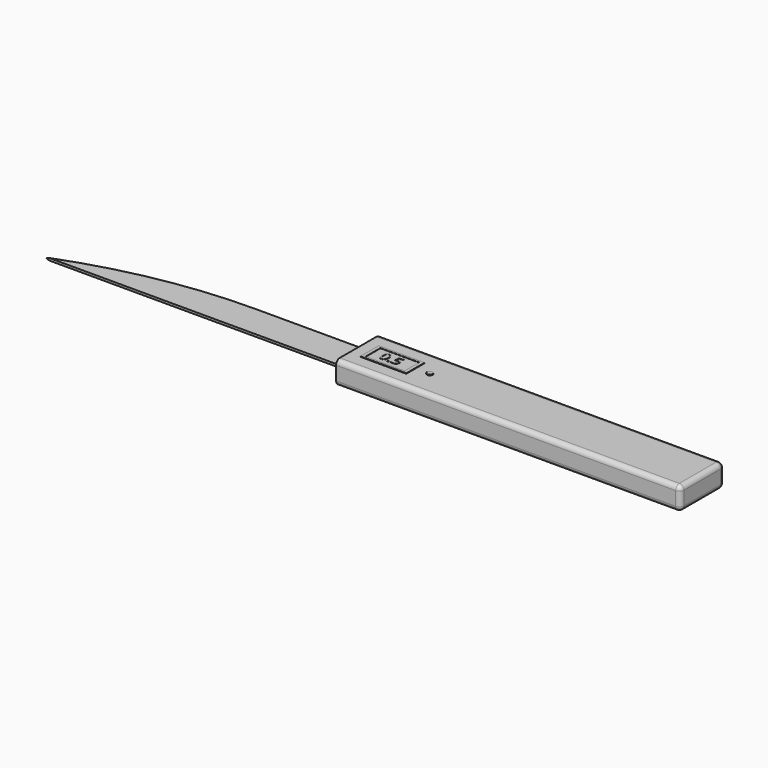
from build123d import *

# Parameters (mm, degrees)
F0_W          = 190.5
F0_H          = 30.48
F1_DEPTH      = 6.35
F1_DEPTH_BACK = 6.35
F3_DEPTH      = 0.635
F3_DEPTH_BACK = 0.635
F4_R          = 2.54
F5_SIZE       = 0.63499
F6_W          = 25.4
F6_H          = 12.7
F7_DEPTH      = 0.254
F8_R          = 1.5875
F9_DEPTH      = 0.381
F10_R         = 0.127
F11_W         = 21.59
F11_H         = 10.16
F12_DEPTH     = 0.127
F13_TEXT_SIZE = 7.8455061343
F14_DEPTH     = 0.127


# Not quite as in the source:
# - a fillet or chamfer is up to 0.001 mm smaller than in the source, because OpenCascade refuses the exact size
# - Text() gives the source's letters only with a copy of the font that has no kerning and outlines rounded to 1/6400 em; it was checked with that copy


with BuildPart() as f1:
    # F0 (on Top) → F1 (new body, two sides)
    with BuildSketch(Plane.XY) as f1_sk:
        with Locations((95.25, 0)):
            Rectangle(F0_W, F0_H)
    extrude(amount=F1_DEPTH)
    extrude(f1_sk.sketch, amount=-F1_DEPTH_BACK)

    # F4
    f4_edges = [f1.edges().sort_by_distance(p)[0] for p in [
        (95.25, -15.24, 6.35),
        (95.25, -15.24, -6.35),
        (190.5, -15.24, 0),
        (190.5, 15.24, 0),
        (95.25, 15.24, 6.35),
        (190.5, 0, -6.35),
        (95.25, 15.24, -6.35),
        (190.5, 0, 6.35),
    ]]
    fillet(f4_edges, radius=F4_R)

    # F6 (on face) → F7 (join)
    with BuildSketch(Plane.XY.offset(6.35)):
        with Locations((19.05, 0)):
            Rectangle(F6_W, F6_H)
    extrude(amount=F7_DEPTH)

    # F11 (on face) → F12 (cut)
    with BuildSketch(Plane.XY.offset(6.604)):
        with Locations((19.05, 0)):
            Rectangle(F11_W, F11_H)
    extrude(amount=-F12_DEPTH, mode=Mode.SUBTRACT)


with BuildPart() as f3:
    # F2 (on Top) → F3 (new body, two sides)
    with BuildSketch(Plane.XY) as f3_sk:
        with BuildLine():
            Line((0, -9.525), (0, 9.525))
            Line((0, 9.525), (-63.5, 9.525))
            ThreePointArc((-63.5, 9.525), (-115.1852553926, 4.721362094), (-165.1, -9.525))
            Line((-165.1, -9.525), (0, -9.525))
        make_face()
    extrude(amount=F3_DEPTH)
    extrude(f3_sk.sketch, amount=-F3_DEPTH_BACK)

    # F5 (size 0.635 in the source; OpenCascade refuses exactly that, so slightly less here)
    f5_edges = [f3.edges().sort_by_distance(p)[0] for p in [
        (-115.185255, 4.721362, 0.635),
        (-115.185255, 4.721362, -0.635),
        (-31.75, 9.525, -0.635),
        (-31.75, 9.525, 0.635),
        (-63.5, 9.525, 0),
        (0, 9.525, 0),
    ]]
    chamfer(f5_edges, length=F5_SIZE)


with BuildPart() as f9:
    # F8 (on face) → F9 (new body)
    with BuildSketch(Plane.XY.offset(6.35)):
        with Locations((39.6875, 0)):
            Circle(F8_R)
    extrude(amount=F9_DEPTH)

    # F10
    f10_edges = [f9.edges().sort_by_distance(p)[0] for p in [
        (38.1, 0, 6.731),
    ]]
    fillet(f10_edges, radius=F10_R)


with BuildPart() as f14:
    # F13 (on face) → F14 (new body)
    with BuildSketch(Plane.XY.offset(6.477)):
        with Locations((12.7, -2.4737644167)):
            Text('0.5', F13_TEXT_SIZE, font='Open Sans', text_align=(TextAlign.LEFT, TextAlign.BOTTOM))
    extrude(amount=F14_DEPTH)


solid = Compound([f1.part, f3.part, f9.part, f14.part])
